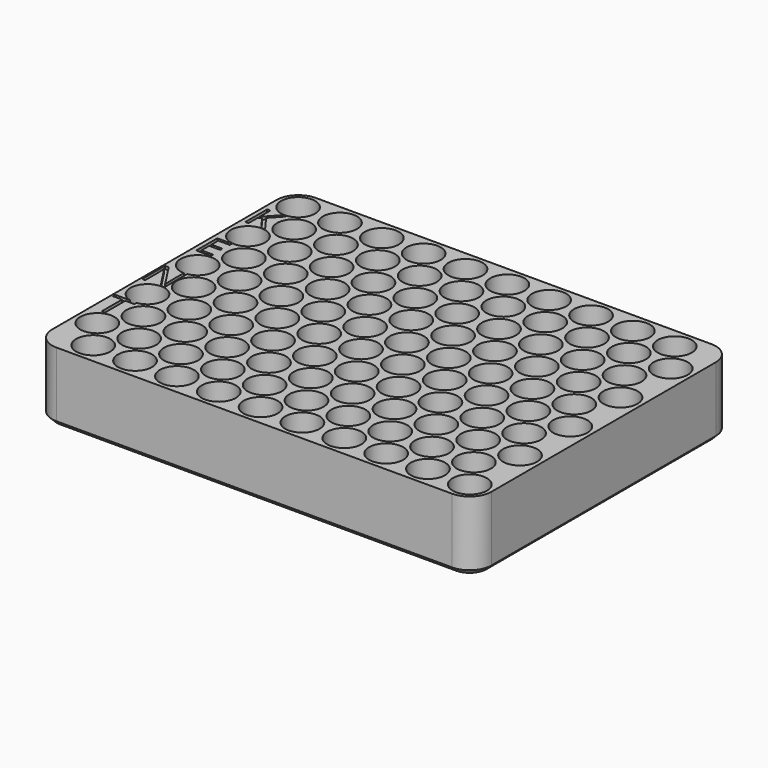
from build123d import *

# Parameters (mm, degrees)
F0_R           = 6.223
F0_R_2         = 3.81
F1_DEPTH       = 5.08
F2_DEPTH       = 20.32
F3_R           = 7.971733183
F4_SIZE        = 1.778
F6_TEXT_SIZE   = 13.9941047463
F6_TEXT_SIZE_2 = 13.4449710863
F6_TEXT_SIZE_3 = 14.5336891162
F6_TEXT_SIZE_4 = 14.5736874806
F7_DEPTH       = 26.4414


# Not quite as in the source:
# - Text() gives the source's letters only with a copy of the font that has no kerning and outlines rounded to 1/6400 em; it was checked with that copy


with BuildPart() as f1:
    # F0 (on Top) → F1 (new body)
    with BuildSketch(Plane.XY):
        Polygon((83.8223695755, 76.2), (76.2, 76.2), (-76.2, 76.2), (-76.2, -41.8424616723), (-60.9797692195, -41.8424616723), (-44.3818755448, -41.8424616723), (51.2277148664, -41.8424616723), (60.9402307805, -41.8424616723), (83.8223695755, -41.8424616723), align=None)
        with Locations((-60.9797692195, -34.2224616723)):
            Circle(F0_R, mode=Mode.SUBTRACT)
        with Locations((-45.7397692195, -34.2224616723)):
            Circle(F0_R, mode=Mode.SUBTRACT)
        with Locations((-68.58, -22.86)):
            Circle(F0_R, mode=Mode.SUBTRACT)
        with Locations((-53.34, -22.86)):
            Circle(F0_R, mode=Mode.SUBTRACT)
        with Locations((-38.1, -22.86)):
            Circle(F0_R, mode=Mode.SUBTRACT)
        with Locations((-30.4997692195, -34.2224616723)):
            Circle(F0_R, mode=Mode.SUBTRACT)
        with Locations((-15.2597692195, -34.2224616723)):
            Circle(F0_R, mode=Mode.SUBTRACT)
        with Locations((-0.0197692195, -34.2224616723)):
            Circle(F0_R, mode=Mode.SUBTRACT)
        with Locations((-22.86, -22.86)):
            Circle(F0_R, mode=Mode.SUBTRACT)
        with Locations((-7.62, -22.86)):
            Circle(F0_R, mode=Mode.SUBTRACT)
        with Locations((-60.9732693728, -11.3624625963)):
            Circle(F0_R, mode=Mode.SUBTRACT)
        with Locations((-68.58, 0)):
            Circle(F0_R, mode=Mode.SUBTRACT)
        with Locations((-45.7332693728, -11.3624625963)):
            Circle(F0_R, mode=Mode.SUBTRACT)
        with Locations((-53.34, 0)):
            Circle(F0_R, mode=Mode.SUBTRACT)
        with Locations((-38.1, 0)):
            Circle(F0_R, mode=Mode.SUBTRACT)
        with Locations((-60.9667695262, 11.4975364796)):
            Circle(F0_R, mode=Mode.SUBTRACT)
        with Locations((-45.7267695262, 11.4975364796)):
            Circle(F0_R, mode=Mode.SUBTRACT)
        with Locations((-30.4932693728, -11.3624625963)):
            Circle(F0_R, mode=Mode.SUBTRACT)
        with Locations((-22.86, 0)):
            Circle(F0_R, mode=Mode.SUBTRACT)
        with Locations((-15.2532693728, -11.3624625963)):
            Circle(F0_R, mode=Mode.SUBTRACT)
        with Locations((-0.0132693728, -11.3624625963)):
            Circle(F0_R, mode=Mode.SUBTRACT)
        with Locations((-7.62, 0)):
            Circle(F0_R, mode=Mode.SUBTRACT)
        with Locations((-30.4867695262, 11.4975364796)):
            Circle(F0_R, mode=Mode.SUBTRACT)
        with Locations((-15.2467695262, 11.4975364796)):
            Circle(F0_R, mode=Mode.SUBTRACT)
        with Locations((-0.0067695262, 11.4975364796)):
            Circle(F0_R, mode=Mode.SUBTRACT)
        with Locations((15.2202307805, -34.2224616723)):
            Circle(F0_R, mode=Mode.SUBTRACT)
        with Locations((30.4602307805, -34.2224616723)):
            Circle(F0_R, mode=Mode.SUBTRACT)
        with Locations((7.62, -22.86)):
            Circle(F0_R, mode=Mode.SUBTRACT)
        with Locations((22.86, -22.86)):
            Circle(F0_R, mode=Mode.SUBTRACT)
        with Locations((38.1, -22.86)):
            Circle(F0_R, mode=Mode.SUBTRACT)
        with Locations((45.7002307805, -34.2224616723)):
            Circle(F0_R, mode=Mode.SUBTRACT)
        with Locations((60.9402307805, -34.2224616723)):
            Circle(F0_R, mode=Mode.SUBTRACT)
        with Locations((76.1802307805, -34.2224616723)):
            Circle(F0_R, mode=Mode.SUBTRACT)
        with Locations((53.34, -22.86)):
            Circle(F0_R, mode=Mode.SUBTRACT)
        with Locations((68.58, -22.86)):
            Circle(F0_R, mode=Mode.SUBTRACT)
        with Locations((15.2267306272, -11.3624625963)):
            Circle(F0_R, mode=Mode.SUBTRACT)
        with Locations((7.62, 0)):
            Circle(F0_R, mode=Mode.SUBTRACT)
        with Locations((22.86, 0)):
            Circle(F0_R, mode=Mode.SUBTRACT)
        with Locations((30.4667306272, -11.3624625963)):
            Circle(F0_R, mode=Mode.SUBTRACT)
        with Locations((38.1, 0)):
            Circle(F0_R, mode=Mode.SUBTRACT)
        with Locations((15.2332304738, 11.4975364796)):
            Circle(F0_R, mode=Mode.SUBTRACT)
        with Locations((30.4732304738, 11.4975364796)):
            Circle(F0_R, mode=Mode.SUBTRACT)
        with Locations((45.7067306272, -11.3624625963)):
            Circle(F0_R, mode=Mode.SUBTRACT)
        with Locations((60.9467306272, -11.3624625963)):
            Circle(F0_R, mode=Mode.SUBTRACT)
        with Locations((53.34, 0)):
            Circle(F0_R, mode=Mode.SUBTRACT)
        with Locations((76.1867306272, -11.3624625963)):
            Circle(F0_R, mode=Mode.SUBTRACT)
        with Locations((68.58, 0)):
            Circle(F0_R, mode=Mode.SUBTRACT)
        with Locations((45.7132304738, 11.4975364796)):
            Circle(F0_R, mode=Mode.SUBTRACT)
        with Locations((60.9532304738, 11.4975364796)):
            Circle(F0_R, mode=Mode.SUBTRACT)
        with Locations((76.1932304738, 11.4975364796)):
            Circle(F0_R, mode=Mode.SUBTRACT)
        with Locations((-68.58, 22.86)):
            Circle(F0_R, mode=Mode.SUBTRACT)
        with Locations((-53.34, 22.86)):
            Circle(F0_R, mode=Mode.SUBTRACT)
        with Locations((-38.1, 22.86)):
            Circle(F0_R, mode=Mode.SUBTRACT)
        with Locations((-60.9602696795, 34.3575355556)):
            Circle(F0_R, mode=Mode.SUBTRACT)
        with Locations((-68.58, 45.72)):
            Circle(F0_R, mode=Mode.SUBTRACT)
        with Locations((-45.7202696795, 34.3575355556)):
            Circle(F0_R, mode=Mode.SUBTRACT)
        with Locations((-53.34, 45.72)):
            Circle(F0_R, mode=Mode.SUBTRACT)
        with Locations((-38.1, 45.72)):
            Circle(F0_R, mode=Mode.SUBTRACT)
        with Locations((-22.86, 22.86)):
            Circle(F0_R, mode=Mode.SUBTRACT)
        with Locations((-7.62, 22.86)):
            Circle(F0_R, mode=Mode.SUBTRACT)
        with Locations((-30.4802696795, 34.3575355556)):
            Circle(F0_R, mode=Mode.SUBTRACT)
        with Locations((-22.86, 45.72)):
            Circle(F0_R, mode=Mode.SUBTRACT)
        with Locations((-15.2402696795, 34.3575355556)):
            Circle(F0_R, mode=Mode.SUBTRACT)
        with Locations((-0.0002696795, 34.3575355556)):
            Circle(F0_R, mode=Mode.SUBTRACT)
        with Locations((-7.62, 45.72)):
            Circle(F0_R, mode=Mode.SUBTRACT)
        with Locations((-60.9537698328, 57.2175346315)):
            Circle(F0_R, mode=Mode.SUBTRACT)
        with Locations((-45.7137698328, 57.2175346315)):
            Circle(F0_R, mode=Mode.SUBTRACT)
        with Locations((-68.58, 68.58)):
            Circle(F0_R, mode=Mode.SUBTRACT)
        with Locations((-53.34, 68.58)):
            Circle(F0_R, mode=Mode.SUBTRACT)
        with Locations((-38.1, 68.58)):
            Circle(F0_R, mode=Mode.SUBTRACT)
        with Locations((-30.4737698328, 57.2175346315)):
            Circle(F0_R, mode=Mode.SUBTRACT)
        with Locations((-15.2337698328, 57.2175346315)):
            Circle(F0_R, mode=Mode.SUBTRACT)
        with Locations((0.0062301672, 57.2175346315)):
            Circle(F0_R, mode=Mode.SUBTRACT)
        with Locations((-22.86, 68.58)):
            Circle(F0_R, mode=Mode.SUBTRACT)
        with Locations((-7.62, 68.58)):
            Circle(F0_R, mode=Mode.SUBTRACT)
        with Locations((7.62, 22.86)):
            Circle(F0_R, mode=Mode.SUBTRACT)
        with Locations((22.86, 22.86)):
            Circle(F0_R, mode=Mode.SUBTRACT)
        with Locations((38.1, 22.86)):
            Circle(F0_R, mode=Mode.SUBTRACT)
        with Locations((15.2397303205, 34.3575355556)):
            Circle(F0_R, mode=Mode.SUBTRACT)
        with Locations((7.62, 45.72)):
            Circle(F0_R, mode=Mode.SUBTRACT)
        with Locations((22.86, 45.72)):
            Circle(F0_R, mode=Mode.SUBTRACT)
        with Locations((30.4797303205, 34.3575355556)):
            Circle(F0_R, mode=Mode.SUBTRACT)
        with Locations((38.1, 45.72)):
            Circle(F0_R, mode=Mode.SUBTRACT)
        with Locations((53.34, 22.86)):
            Circle(F0_R, mode=Mode.SUBTRACT)
        with Locations((68.58, 22.86)):
            Circle(F0_R, mode=Mode.SUBTRACT)
        with Locations((45.7197303205, 34.3575355556)):
            Circle(F0_R, mode=Mode.SUBTRACT)
        with Locations((60.9597303205, 34.3575355556)):
            Circle(F0_R, mode=Mode.SUBTRACT)
        with Locations((53.34, 45.72)):
            Circle(F0_R, mode=Mode.SUBTRACT)
        with Locations((76.1997303205, 34.3575355556)):
            Circle(F0_R, mode=Mode.SUBTRACT)
        with Locations((68.58, 45.72)):
            Circle(F0_R, mode=Mode.SUBTRACT)
        with Locations((15.2462301672, 57.2175346315)):
            Circle(F0_R, mode=Mode.SUBTRACT)
        with Locations((30.4862301672, 57.2175346315)):
            Circle(F0_R, mode=Mode.SUBTRACT)
        with Locations((7.62, 68.58)):
            Circle(F0_R, mode=Mode.SUBTRACT)
        with Locations((22.86, 68.58)):
            Circle(F0_R, mode=Mode.SUBTRACT)
        with Locations((38.1, 68.58)):
            Circle(F0_R, mode=Mode.SUBTRACT)
        with Locations((45.7262301672, 57.2175346315)):
            Circle(F0_R, mode=Mode.SUBTRACT)
        with Locations((60.9662301672, 57.2175346315)):
            Circle(F0_R, mode=Mode.SUBTRACT)
        with Locations((76.2062301672, 57.2175346315)):
            Circle(F0_R, mode=Mode.SUBTRACT)
        with Locations((53.34, 68.58)):
            Circle(F0_R, mode=Mode.SUBTRACT)
        with Locations((68.58, 68.58)):
            Circle(F0_R, mode=Mode.SUBTRACT)
        with Locations((-30.4932693728, -11.3624625963)):
            Circle(F0_R)
        with Locations((-30.4932693728, -11.3624625963)):
            Circle(F0_R_2, mode=Mode.SUBTRACT)
        with Locations((-38.1, 0)):
            Circle(F0_R)
        with Locations((-38.1, 0)):
            Circle(F0_R_2, mode=Mode.SUBTRACT)
        with Locations((-45.7332693728, -11.3624625963)):
            Circle(F0_R)
        with Locations((-45.7332693728, -11.3624625963)):
            Circle(F0_R_2, mode=Mode.SUBTRACT)
        with Locations((-38.1, -22.86)):
            Circle(F0_R)
        with Locations((-38.1, -22.86)):
            Circle(F0_R_2, mode=Mode.SUBTRACT)
        with Locations((-45.7397692195, -34.2224616723)):
            Circle(F0_R)
        with Locations((-45.7397692195, -34.2224616723)):
            Circle(F0_R_2, mode=Mode.SUBTRACT)
        with Locations((-30.4997692195, -34.2224616723)):
            Circle(F0_R)
        with Locations((-30.4997692195, -34.2224616723)):
            Circle(F0_R_2, mode=Mode.SUBTRACT)
        with Locations((-22.86, -22.86)):
            Circle(F0_R)
        with Locations((-22.86, -22.86)):
            Circle(F0_R_2, mode=Mode.SUBTRACT)
        with Locations((-15.2532693728, -11.3624625963)):
            Circle(F0_R)
        with Locations((-15.2532693728, -11.3624625963)):
            Circle(F0_R_2, mode=Mode.SUBTRACT)
        with Locations((-22.86, 0)):
            Circle(F0_R)
        with Locations((-22.86, 0)):
            Circle(F0_R_2, mode=Mode.SUBTRACT)
        with Locations((-53.34, 0)):
            Circle(F0_R)
        with Locations((-53.34, 0)):
            Circle(F0_R_2, mode=Mode.SUBTRACT)
        with Locations((-60.9732693728, -11.3624625963)):
            Circle(F0_R)
        with Locations((-60.9732693728, -11.3624625963)):
            Circle(F0_R_2, mode=Mode.SUBTRACT)
        with Locations((-53.34, -22.86)):
            Circle(F0_R)
        with Locations((-53.34, -22.86)):
            Circle(F0_R_2, mode=Mode.SUBTRACT)
        with Locations((-60.9797692195, -34.2224616723)):
            Circle(F0_R)
        with Locations((-60.9797692195, -34.2224616723)):
            Circle(F0_R_2, mode=Mode.SUBTRACT)
        with Locations((-68.58, -22.86)):
            Circle(F0_R)
        with Locations((-68.58, -22.86)):
            Circle(F0_R_2, mode=Mode.SUBTRACT)
        with Locations((-68.58, 0)):
            Circle(F0_R)
        with Locations((-68.58, 0)):
            Circle(F0_R_2, mode=Mode.SUBTRACT)
        with Locations((-7.62, 0)):
            Circle(F0_R)
        with Locations((-7.62, 0)):
            Circle(F0_R_2, mode=Mode.SUBTRACT)
        with Locations((-0.0132693728, -11.3624625963)):
            Circle(F0_R)
        with Locations((-0.0132693728, -11.3624625963)):
            Circle(F0_R_2, mode=Mode.SUBTRACT)
        with Locations((-7.62, -22.86)):
            Circle(F0_R)
        with Locations((-7.62, -22.86)):
            Circle(F0_R_2, mode=Mode.SUBTRACT)
        with Locations((-15.2597692195, -34.2224616723)):
            Circle(F0_R)
        with Locations((-15.2597692195, -34.2224616723)):
            Circle(F0_R_2, mode=Mode.SUBTRACT)
        with Locations((-0.0197692195, -34.2224616723)):
            Circle(F0_R)
        with Locations((-0.0197692195, -34.2224616723)):
            Circle(F0_R_2, mode=Mode.SUBTRACT)
        with Locations((7.62, -22.86)):
            Circle(F0_R)
        with Locations((7.62, -22.86)):
            Circle(F0_R_2, mode=Mode.SUBTRACT)
        with Locations((15.2202307805, -34.2224616723)):
            Circle(F0_R)
        with Locations((15.2202307805, -34.2224616723)):
            Circle(F0_R_2, mode=Mode.SUBTRACT)
        with Locations((22.86, -22.86)):
            Circle(F0_R)
        with Locations((22.86, -22.86)):
            Circle(F0_R_2, mode=Mode.SUBTRACT)
        with Locations((15.2267306272, -11.3624625963)):
            Circle(F0_R)
        with Locations((15.2267306272, -11.3624625963)):
            Circle(F0_R_2, mode=Mode.SUBTRACT)
        with Locations((7.62, 0)):
            Circle(F0_R)
        with Locations((7.62, 0)):
            Circle(F0_R_2, mode=Mode.SUBTRACT)
        with Locations((-15.2467695262, 11.4975364796)):
            Circle(F0_R)
        with Locations((-15.2467695262, 11.4975364796)):
            Circle(F0_R_2, mode=Mode.SUBTRACT)
        with Locations((-30.4867695262, 11.4975364796)):
            Circle(F0_R)
        with Locations((-30.4867695262, 11.4975364796)):
            Circle(F0_R_2, mode=Mode.SUBTRACT)
        with Locations((-45.7267695262, 11.4975364796)):
            Circle(F0_R)
        with Locations((-45.7267695262, 11.4975364796)):
            Circle(F0_R_2, mode=Mode.SUBTRACT)
        with Locations((-60.9667695262, 11.4975364796)):
            Circle(F0_R)
        with Locations((-60.9667695262, 11.4975364796)):
            Circle(F0_R_2, mode=Mode.SUBTRACT)
        with Locations((-53.34, 22.86)):
            Circle(F0_R)
        with Locations((-53.34, 22.86)):
            Circle(F0_R_2, mode=Mode.SUBTRACT)
        with Locations((-38.1, 22.86)):
            Circle(F0_R)
        with Locations((-38.1, 22.86)):
            Circle(F0_R_2, mode=Mode.SUBTRACT)
        with Locations((-22.86, 22.86)):
            Circle(F0_R)
        with Locations((-22.86, 22.86)):
            Circle(F0_R_2, mode=Mode.SUBTRACT)
        with Locations((-7.62, 22.86)):
            Circle(F0_R)
        with Locations((-7.62, 22.86)):
            Circle(F0_R_2, mode=Mode.SUBTRACT)
        with Locations((-0.0067695262, 11.4975364796)):
            Circle(F0_R)
        with Locations((-0.0067695262, 11.4975364796)):
            Circle(F0_R_2, mode=Mode.SUBTRACT)
        with Locations((15.2332304738, 11.4975364796)):
            Circle(F0_R)
        with Locations((15.2332304738, 11.4975364796)):
            Circle(F0_R_2, mode=Mode.SUBTRACT)
        with Locations((76.1802307805, -34.2224616723)):
            Circle(F0_R)
        with Locations((76.1802307805, -34.2224616723)):
            Circle(F0_R_2, mode=Mode.SUBTRACT)
        with Locations((60.9402307805, -34.2224616723)):
            Circle(F0_R)
        with Locations((60.9402307805, -34.2224616723)):
            Circle(F0_R_2, mode=Mode.SUBTRACT)
        with Locations((45.7002307805, -34.2224616723)):
            Circle(F0_R)
        with Locations((45.7002307805, -34.2224616723)):
            Circle(F0_R_2, mode=Mode.SUBTRACT)
        with Locations((30.4602307805, -34.2224616723)):
            Circle(F0_R)
        with Locations((30.4602307805, -34.2224616723)):
            Circle(F0_R_2, mode=Mode.SUBTRACT)
        with Locations((38.1, -22.86)):
            Circle(F0_R)
        with Locations((38.1, -22.86)):
            Circle(F0_R_2, mode=Mode.SUBTRACT)
        with Locations((53.34, -22.86)):
            Circle(F0_R)
        with Locations((53.34, -22.86)):
            Circle(F0_R_2, mode=Mode.SUBTRACT)
        with Locations((68.58, -22.86)):
            Circle(F0_R)
        with Locations((68.58, -22.86)):
            Circle(F0_R_2, mode=Mode.SUBTRACT)
        with Locations((60.9467306272, -11.3624625963)):
            Circle(F0_R)
        with Locations((60.9467306272, -11.3624625963)):
            Circle(F0_R_2, mode=Mode.SUBTRACT)
        with Locations((76.1867306272, -11.3624625963)):
            Circle(F0_R)
        with Locations((76.1867306272, -11.3624625963)):
            Circle(F0_R_2, mode=Mode.SUBTRACT)
        with Locations((45.7067306272, -11.3624625963)):
            Circle(F0_R)
        with Locations((45.7067306272, -11.3624625963)):
            Circle(F0_R_2, mode=Mode.SUBTRACT)
        with Locations((30.4667306272, -11.3624625963)):
            Circle(F0_R)
        with Locations((30.4667306272, -11.3624625963)):
            Circle(F0_R_2, mode=Mode.SUBTRACT)
        with Locations((38.1, 0)):
            Circle(F0_R)
        with Locations((38.1, 0)):
            Circle(F0_R_2, mode=Mode.SUBTRACT)
        with Locations((22.86, 0)):
            Circle(F0_R)
        with Locations((22.86, 0)):
            Circle(F0_R_2, mode=Mode.SUBTRACT)
        with Locations((53.34, 0)):
            Circle(F0_R)
        with Locations((53.34, 0)):
            Circle(F0_R_2, mode=Mode.SUBTRACT)
        with Locations((68.58, 0)):
            Circle(F0_R)
        with Locations((68.58, 0)):
            Circle(F0_R_2, mode=Mode.SUBTRACT)
        with Locations((76.1932304738, 11.4975364796)):
            Circle(F0_R)
        with Locations((76.1932304738, 11.4975364796)):
            Circle(F0_R_2, mode=Mode.SUBTRACT)
        with Locations((60.9532304738, 11.4975364796)):
            Circle(F0_R)
        with Locations((60.9532304738, 11.4975364796)):
            Circle(F0_R_2, mode=Mode.SUBTRACT)
        with Locations((45.7132304738, 11.4975364796)):
            Circle(F0_R)
        with Locations((45.7132304738, 11.4975364796)):
            Circle(F0_R_2, mode=Mode.SUBTRACT)
        with Locations((30.4732304738, 11.4975364796)):
            Circle(F0_R)
        with Locations((30.4732304738, 11.4975364796)):
            Circle(F0_R_2, mode=Mode.SUBTRACT)
        with Locations((22.86, 22.86)):
            Circle(F0_R)
        with Locations((22.86, 22.86)):
            Circle(F0_R_2, mode=Mode.SUBTRACT)
        with Locations((38.1, 22.86)):
            Circle(F0_R)
        with Locations((38.1, 22.86)):
            Circle(F0_R_2, mode=Mode.SUBTRACT)
        with Locations((7.62, 22.86)):
            Circle(F0_R)
        with Locations((7.62, 22.86)):
            Circle(F0_R_2, mode=Mode.SUBTRACT)
        with Locations((15.2397303205, 34.3575355556)):
            Circle(F0_R)
        with Locations((15.2397303205, 34.3575355556)):
            Circle(F0_R_2, mode=Mode.SUBTRACT)
        with Locations((30.4797303205, 34.3575355556)):
            Circle(F0_R)
        with Locations((30.4797303205, 34.3575355556)):
            Circle(F0_R_2, mode=Mode.SUBTRACT)
        with Locations((-0.0002696795, 34.3575355556)):
            Circle(F0_R)
        with Locations((-0.0002696795, 34.3575355556)):
            Circle(F0_R_2, mode=Mode.SUBTRACT)
        with Locations((-15.2402696795, 34.3575355556)):
            Circle(F0_R)
        with Locations((-15.2402696795, 34.3575355556)):
            Circle(F0_R_2, mode=Mode.SUBTRACT)
        with Locations((-45.7137698328, 57.2175346315)):
            Circle(F0_R)
        with Locations((-45.7137698328, 57.2175346315)):
            Circle(F0_R_2, mode=Mode.SUBTRACT)
        with Locations((-60.9537698328, 57.2175346315)):
            Circle(F0_R)
        with Locations((-60.9537698328, 57.2175346315)):
            Circle(F0_R_2, mode=Mode.SUBTRACT)
        with Locations((-68.58, 45.72)):
            Circle(F0_R)
        with Locations((-68.58, 45.72)):
            Circle(F0_R_2, mode=Mode.SUBTRACT)
        with Locations((-53.34, 45.72)):
            Circle(F0_R)
        with Locations((-53.34, 45.72)):
            Circle(F0_R_2, mode=Mode.SUBTRACT)
        with Locations((-68.58, 22.86)):
            Circle(F0_R)
        with Locations((-68.58, 22.86)):
            Circle(F0_R_2, mode=Mode.SUBTRACT)
        with Locations((-60.9602696795, 34.3575355556)):
            Circle(F0_R)
        with Locations((-60.9602696795, 34.3575355556)):
            Circle(F0_R_2, mode=Mode.SUBTRACT)
        with Locations((-45.7202696795, 34.3575355556)):
            Circle(F0_R)
        with Locations((-45.7202696795, 34.3575355556)):
            Circle(F0_R_2, mode=Mode.SUBTRACT)
        with Locations((-30.4802696795, 34.3575355556)):
            Circle(F0_R)
        with Locations((-30.4802696795, 34.3575355556)):
            Circle(F0_R_2, mode=Mode.SUBTRACT)
        with Locations((-38.1, 45.72)):
            Circle(F0_R)
        with Locations((-38.1, 45.72)):
            Circle(F0_R_2, mode=Mode.SUBTRACT)
        with Locations((-22.86, 45.72)):
            Circle(F0_R)
        with Locations((-22.86, 45.72)):
            Circle(F0_R_2, mode=Mode.SUBTRACT)
        with Locations((-30.4737698328, 57.2175346315)):
            Circle(F0_R)
        with Locations((-30.4737698328, 57.2175346315)):
            Circle(F0_R_2, mode=Mode.SUBTRACT)
        with Locations((-15.2337698328, 57.2175346315)):
            Circle(F0_R)
        with Locations((-15.2337698328, 57.2175346315)):
            Circle(F0_R_2, mode=Mode.SUBTRACT)
        with Locations((0.0062301672, 57.2175346315)):
            Circle(F0_R)
        with Locations((0.0062301672, 57.2175346315)):
            Circle(F0_R_2, mode=Mode.SUBTRACT)
        with Locations((-7.62, 45.72)):
            Circle(F0_R)
        with Locations((-7.62, 45.72)):
            Circle(F0_R_2, mode=Mode.SUBTRACT)
        with Locations((7.62, 45.72)):
            Circle(F0_R)
        with Locations((7.62, 45.72)):
            Circle(F0_R_2, mode=Mode.SUBTRACT)
        with Locations((15.2462301672, 57.2175346315)):
            Circle(F0_R)
        with Locations((15.2462301672, 57.2175346315)):
            Circle(F0_R_2, mode=Mode.SUBTRACT)
        with Locations((7.62, 68.58)):
            Circle(F0_R)
        with Locations((7.62, 68.58)):
            Circle(F0_R_2, mode=Mode.SUBTRACT)
        with Locations((-22.86, 68.58)):
            Circle(F0_R)
        with Locations((-22.86, 68.58)):
            Circle(F0_R_2, mode=Mode.SUBTRACT)
        with Locations((-38.1, 68.58)):
            Circle(F0_R)
        with Locations((-38.1, 68.58)):
            Circle(F0_R_2, mode=Mode.SUBTRACT)
        with Locations((-7.62, 68.58)):
            Circle(F0_R)
        with Locations((-7.62, 68.58)):
            Circle(F0_R_2, mode=Mode.SUBTRACT)
        with Locations((22.86, 68.58)):
            Circle(F0_R)
        with Locations((22.86, 68.58)):
            Circle(F0_R_2, mode=Mode.SUBTRACT)
        with Locations((-53.34, 68.58)):
            Circle(F0_R)
        with Locations((-53.34, 68.58)):
            Circle(F0_R_2, mode=Mode.SUBTRACT)
        with Locations((-68.58, 68.58)):
            Circle(F0_R)
        with Locations((-68.58, 68.58)):
            Circle(F0_R_2, mode=Mode.SUBTRACT)
        with Locations((30.4862301672, 57.2175346315)):
            Circle(F0_R)
        with Locations((30.4862301672, 57.2175346315)):
            Circle(F0_R_2, mode=Mode.SUBTRACT)
        with Locations((22.86, 45.72)):
            Circle(F0_R)
        with Locations((22.86, 45.72)):
            Circle(F0_R_2, mode=Mode.SUBTRACT)
        with Locations((38.1, 45.72)):
            Circle(F0_R)
        with Locations((38.1, 45.72)):
            Circle(F0_R_2, mode=Mode.SUBTRACT)
        with Locations((45.7197303205, 34.3575355556)):
            Circle(F0_R)
        with Locations((45.7197303205, 34.3575355556)):
            Circle(F0_R_2, mode=Mode.SUBTRACT)
        with Locations((53.34, 22.86)):
            Circle(F0_R)
        with Locations((53.34, 22.86)):
            Circle(F0_R_2, mode=Mode.SUBTRACT)
        with Locations((45.7262301672, 57.2175346315)):
            Circle(F0_R)
        with Locations((45.7262301672, 57.2175346315)):
            Circle(F0_R_2, mode=Mode.SUBTRACT)
        with Locations((38.1, 68.58)):
            Circle(F0_R)
        with Locations((38.1, 68.58)):
            Circle(F0_R_2, mode=Mode.SUBTRACT)
        with Locations((53.34, 68.58)):
            Circle(F0_R)
        with Locations((53.34, 68.58)):
            Circle(F0_R_2, mode=Mode.SUBTRACT)
        with Locations((68.58, 22.86)):
            Circle(F0_R)
        with Locations((68.58, 22.86)):
            Circle(F0_R_2, mode=Mode.SUBTRACT)
        with Locations((76.1997303205, 34.3575355556)):
            Circle(F0_R)
        with Locations((76.1997303205, 34.3575355556)):
            Circle(F0_R_2, mode=Mode.SUBTRACT)
        with Locations((60.9597303205, 34.3575355556)):
            Circle(F0_R)
        with Locations((60.9597303205, 34.3575355556)):
            Circle(F0_R_2, mode=Mode.SUBTRACT)
        with Locations((53.34, 45.72)):
            Circle(F0_R)
        with Locations((53.34, 45.72)):
            Circle(F0_R_2, mode=Mode.SUBTRACT)
        with Locations((68.58, 45.72)):
            Circle(F0_R)
        with Locations((68.58, 45.72)):
            Circle(F0_R_2, mode=Mode.SUBTRACT)
        with Locations((60.9662301672, 57.2175346315)):
            Circle(F0_R)
        with Locations((60.9662301672, 57.2175346315)):
            Circle(F0_R_2, mode=Mode.SUBTRACT)
        with Locations((76.2062301672, 57.2175346315)):
            Circle(F0_R)
        with Locations((76.2062301672, 57.2175346315)):
            Circle(F0_R_2, mode=Mode.SUBTRACT)
        with Locations((68.58, 68.58)):
            Circle(F0_R)
        with Locations((68.58, 68.58)):
            Circle(F0_R_2, mode=Mode.SUBTRACT)
    extrude(amount=-F1_DEPTH)

    # F0 (on Top) → F2 (join)
    with BuildSketch(Plane.XY):
        Polygon((83.8223695755, 76.2), (76.2, 76.2), (-76.2, 76.2), (-76.2, -41.8424616723), (-60.9797692195, -41.8424616723), (-44.3818755448, -41.8424616723), (51.2277148664, -41.8424616723), (60.9402307805, -41.8424616723), (83.8223695755, -41.8424616723), align=None)
        with Locations((-60.9797692195, -34.2224616723)):
            Circle(F0_R, mode=Mode.SUBTRACT)
        with Locations((-45.7397692195, -34.2224616723)):
            Circle(F0_R, mode=Mode.SUBTRACT)
        with Locations((-68.58, -22.86)):
            Circle(F0_R, mode=Mode.SUBTRACT)
        with Locations((-53.34, -22.86)):
            Circle(F0_R, mode=Mode.SUBTRACT)
        with Locations((-38.1, -22.86)):
            Circle(F0_R, mode=Mode.SUBTRACT)
        with Locations((-30.4997692195, -34.2224616723)):
            Circle(F0_R, mode=Mode.SUBTRACT)
        with Locations((-15.2597692195, -34.2224616723)):
            Circle(F0_R, mode=Mode.SUBTRACT)
        with Locations((-0.0197692195, -34.2224616723)):
            Circle(F0_R, mode=Mode.SUBTRACT)
        with Locations((-22.86, -22.86)):
            Circle(F0_R, mode=Mode.SUBTRACT)
        with Locations((-7.62, -22.86)):
            Circle(F0_R, mode=Mode.SUBTRACT)
        with Locations((-60.9732693728, -11.3624625963)):
            Circle(F0_R, mode=Mode.SUBTRACT)
        with Locations((-68.58, 0)):
            Circle(F0_R, mode=Mode.SUBTRACT)
        with Locations((-45.7332693728, -11.3624625963)):
            Circle(F0_R, mode=Mode.SUBTRACT)
        with Locations((-53.34, 0)):
            Circle(F0_R, mode=Mode.SUBTRACT)
        with Locations((-38.1, 0)):
            Circle(F0_R, mode=Mode.SUBTRACT)
        with Locations((-60.9667695262, 11.4975364796)):
            Circle(F0_R, mode=Mode.SUBTRACT)
        with Locations((-45.7267695262, 11.4975364796)):
            Circle(F0_R, mode=Mode.SUBTRACT)
        with Locations((-30.4932693728, -11.3624625963)):
            Circle(F0_R, mode=Mode.SUBTRACT)
        with Locations((-22.86, 0)):
            Circle(F0_R, mode=Mode.SUBTRACT)
        with Locations((-15.2532693728, -11.3624625963)):
            Circle(F0_R, mode=Mode.SUBTRACT)
        with Locations((-0.0132693728, -11.3624625963)):
            Circle(F0_R, mode=Mode.SUBTRACT)
        with Locations((-7.62, 0)):
            Circle(F0_R, mode=Mode.SUBTRACT)
        with Locations((-30.4867695262, 11.4975364796)):
            Circle(F0_R, mode=Mode.SUBTRACT)
        with Locations((-15.2467695262, 11.4975364796)):
            Circle(F0_R, mode=Mode.SUBTRACT)
        with Locations((-0.0067695262, 11.4975364796)):
            Circle(F0_R, mode=Mode.SUBTRACT)
        with Locations((15.2202307805, -34.2224616723)):
            Circle(F0_R, mode=Mode.SUBTRACT)
        with Locations((30.4602307805, -34.2224616723)):
            Circle(F0_R, mode=Mode.SUBTRACT)
        with Locations((7.62, -22.86)):
            Circle(F0_R, mode=Mode.SUBTRACT)
        with Locations((22.86, -22.86)):
            Circle(F0_R, mode=Mode.SUBTRACT)
        with Locations((38.1, -22.86)):
            Circle(F0_R, mode=Mode.SUBTRACT)
        with Locations((45.7002307805, -34.2224616723)):
            Circle(F0_R, mode=Mode.SUBTRACT)
        with Locations((60.9402307805, -34.2224616723)):
            Circle(F0_R, mode=Mode.SUBTRACT)
        with Locations((76.1802307805, -34.2224616723)):
            Circle(F0_R, mode=Mode.SUBTRACT)
        with Locations((53.34, -22.86)):
            Circle(F0_R, mode=Mode.SUBTRACT)
        with Locations((68.58, -22.86)):
            Circle(F0_R, mode=Mode.SUBTRACT)
        with Locations((15.2267306272, -11.3624625963)):
            Circle(F0_R, mode=Mode.SUBTRACT)
        with Locations((7.62, 0)):
            Circle(F0_R, mode=Mode.SUBTRACT)
        with Locations((22.86, 0)):
            Circle(F0_R, mode=Mode.SUBTRACT)
        with Locations((30.4667306272, -11.3624625963)):
            Circle(F0_R, mode=Mode.SUBTRACT)
        with Locations((38.1, 0)):
            Circle(F0_R, mode=Mode.SUBTRACT)
        with Locations((15.2332304738, 11.4975364796)):
            Circle(F0_R, mode=Mode.SUBTRACT)
        with Locations((30.4732304738, 11.4975364796)):
            Circle(F0_R, mode=Mode.SUBTRACT)
        with Locations((45.7067306272, -11.3624625963)):
            Circle(F0_R, mode=Mode.SUBTRACT)
        with Locations((60.9467306272, -11.3624625963)):
            Circle(F0_R, mode=Mode.SUBTRACT)
        with Locations((53.34, 0)):
            Circle(F0_R, mode=Mode.SUBTRACT)
        with Locations((76.1867306272, -11.3624625963)):
            Circle(F0_R, mode=Mode.SUBTRACT)
        with Locations((68.58, 0)):
            Circle(F0_R, mode=Mode.SUBTRACT)
        with Locations((45.7132304738, 11.4975364796)):
            Circle(F0_R, mode=Mode.SUBTRACT)
        with Locations((60.9532304738, 11.4975364796)):
            Circle(F0_R, mode=Mode.SUBTRACT)
        with Locations((76.1932304738, 11.4975364796)):
            Circle(F0_R, mode=Mode.SUBTRACT)
        with Locations((-68.58, 22.86)):
            Circle(F0_R, mode=Mode.SUBTRACT)
        with Locations((-53.34, 22.86)):
            Circle(F0_R, mode=Mode.SUBTRACT)
        with Locations((-38.1, 22.86)):
            Circle(F0_R, mode=Mode.SUBTRACT)
        with Locations((-60.9602696795, 34.3575355556)):
            Circle(F0_R, mode=Mode.SUBTRACT)
        with Locations((-68.58, 45.72)):
            Circle(F0_R, mode=Mode.SUBTRACT)
        with Locations((-45.7202696795, 34.3575355556)):
            Circle(F0_R, mode=Mode.SUBTRACT)
        with Locations((-53.34, 45.72)):
            Circle(F0_R, mode=Mode.SUBTRACT)
        with Locations((-38.1, 45.72)):
            Circle(F0_R, mode=Mode.SUBTRACT)
        with Locations((-22.86, 22.86)):
            Circle(F0_R, mode=Mode.SUBTRACT)
        with Locations((-7.62, 22.86)):
            Circle(F0_R, mode=Mode.SUBTRACT)
        with Locations((-30.4802696795, 34.3575355556)):
            Circle(F0_R, mode=Mode.SUBTRACT)
        with Locations((-22.86, 45.72)):
            Circle(F0_R, mode=Mode.SUBTRACT)
        with Locations((-15.2402696795, 34.3575355556)):
            Circle(F0_R, mode=Mode.SUBTRACT)
        with Locations((-0.0002696795, 34.3575355556)):
            Circle(F0_R, mode=Mode.SUBTRACT)
        with Locations((-7.62, 45.72)):
            Circle(F0_R, mode=Mode.SUBTRACT)
        with Locations((-60.9537698328, 57.2175346315)):
            Circle(F0_R, mode=Mode.SUBTRACT)
        with Locations((-45.7137698328, 57.2175346315)):
            Circle(F0_R, mode=Mode.SUBTRACT)
        with Locations((-68.58, 68.58)):
            Circle(F0_R, mode=Mode.SUBTRACT)
        with Locations((-53.34, 68.58)):
            Circle(F0_R, mode=Mode.SUBTRACT)
        with Locations((-38.1, 68.58)):
            Circle(F0_R, mode=Mode.SUBTRACT)
        with Locations((-30.4737698328, 57.2175346315)):
            Circle(F0_R, mode=Mode.SUBTRACT)
        with Locations((-15.2337698328, 57.2175346315)):
            Circle(F0_R, mode=Mode.SUBTRACT)
        with Locations((0.0062301672, 57.2175346315)):
            Circle(F0_R, mode=Mode.SUBTRACT)
        with Locations((-22.86, 68.58)):
            Circle(F0_R, mode=Mode.SUBTRACT)
        with Locations((-7.62, 68.58)):
            Circle(F0_R, mode=Mode.SUBTRACT)
        with Locations((7.62, 22.86)):
            Circle(F0_R, mode=Mode.SUBTRACT)
        with Locations((22.86, 22.86)):
            Circle(F0_R, mode=Mode.SUBTRACT)
        with Locations((38.1, 22.86)):
            Circle(F0_R, mode=Mode.SUBTRACT)
        with Locations((15.2397303205, 34.3575355556)):
            Circle(F0_R, mode=Mode.SUBTRACT)
        with Locations((7.62, 45.72)):
            Circle(F0_R, mode=Mode.SUBTRACT)
        with Locations((22.86, 45.72)):
            Circle(F0_R, mode=Mode.SUBTRACT)
        with Locations((30.4797303205, 34.3575355556)):
            Circle(F0_R, mode=Mode.SUBTRACT)
        with Locations((38.1, 45.72)):
            Circle(F0_R, mode=Mode.SUBTRACT)
        with Locations((53.34, 22.86)):
            Circle(F0_R, mode=Mode.SUBTRACT)
        with Locations((68.58, 22.86)):
            Circle(F0_R, mode=Mode.SUBTRACT)
        with Locations((45.7197303205, 34.3575355556)):
            Circle(F0_R, mode=Mode.SUBTRACT)
        with Locations((60.9597303205, 34.3575355556)):
            Circle(F0_R, mode=Mode.SUBTRACT)
        with Locations((53.34, 45.72)):
            Circle(F0_R, mode=Mode.SUBTRACT)
        with Locations((76.1997303205, 34.3575355556)):
            Circle(F0_R, mode=Mode.SUBTRACT)
        with Locations((68.58, 45.72)):
            Circle(F0_R, mode=Mode.SUBTRACT)
        with Locations((15.2462301672, 57.2175346315)):
            Circle(F0_R, mode=Mode.SUBTRACT)
        with Locations((30.4862301672, 57.2175346315)):
            Circle(F0_R, mode=Mode.SUBTRACT)
        with Locations((7.62, 68.58)):
            Circle(F0_R, mode=Mode.SUBTRACT)
        with Locations((22.86, 68.58)):
            Circle(F0_R, mode=Mode.SUBTRACT)
        with Locations((38.1, 68.58)):
            Circle(F0_R, mode=Mode.SUBTRACT)
        with Locations((45.7262301672, 57.2175346315)):
            Circle(F0_R, mode=Mode.SUBTRACT)
        with Locations((60.9662301672, 57.2175346315)):
            Circle(F0_R, mode=Mode.SUBTRACT)
        with Locations((76.2062301672, 57.2175346315)):
            Circle(F0_R, mode=Mode.SUBTRACT)
        with Locations((53.34, 68.58)):
            Circle(F0_R, mode=Mode.SUBTRACT)
        with Locations((68.58, 68.58)):
            Circle(F0_R, mode=Mode.SUBTRACT)
    extrude(amount=F2_DEPTH)

    # F3
    f3_edges = [f1.edges().sort_by_distance(p)[0] for p in [
        (-76.2, -41.842462, 7.62),
        (83.82237, -41.842462, 7.62),
        (83.82237, 76.2, 7.62),
        (-76.2, 76.2, 7.62),
    ]]
    fillet(f3_edges, radius=F3_R)

    # F4
    f4_edges = [f1.edges().sort_by_distance(p)[0] for p in [
        (-76.2, 17.178769, -5.08),
    ]]
    chamfer(f4_edges, length=F4_SIZE)

    # F6 (on offset) → F7 (cut)
    with BuildSketch(Plane.XY.offset(45.72)):
        with Locations((-76.0100781918, 52.0949624479)):
            Text('K', F6_TEXT_SIZE, font='Open Sans', text_align=(TextAlign.LEFT, TextAlign.BOTTOM))
        with Locations((-75.8973881602, 29.6856090426)):
            Text('E', F6_TEXT_SIZE_2, font='Open Sans', text_align=(TextAlign.LEFT, TextAlign.BOTTOM))
        with Locations((-77.0418867469, 6.357118953)):
            Text('N', F6_TEXT_SIZE_3, font='Open Sans', text_align=(TextAlign.LEFT, TextAlign.BOTTOM))
        with Locations((-75.5862668157, -16.4328441024)):
            Text('T', F6_TEXT_SIZE_4, font='Open Sans', text_align=(TextAlign.LEFT, TextAlign.BOTTOM))
    extrude(amount=-F7_DEPTH, mode=Mode.SUBTRACT)


solid = f1.part
